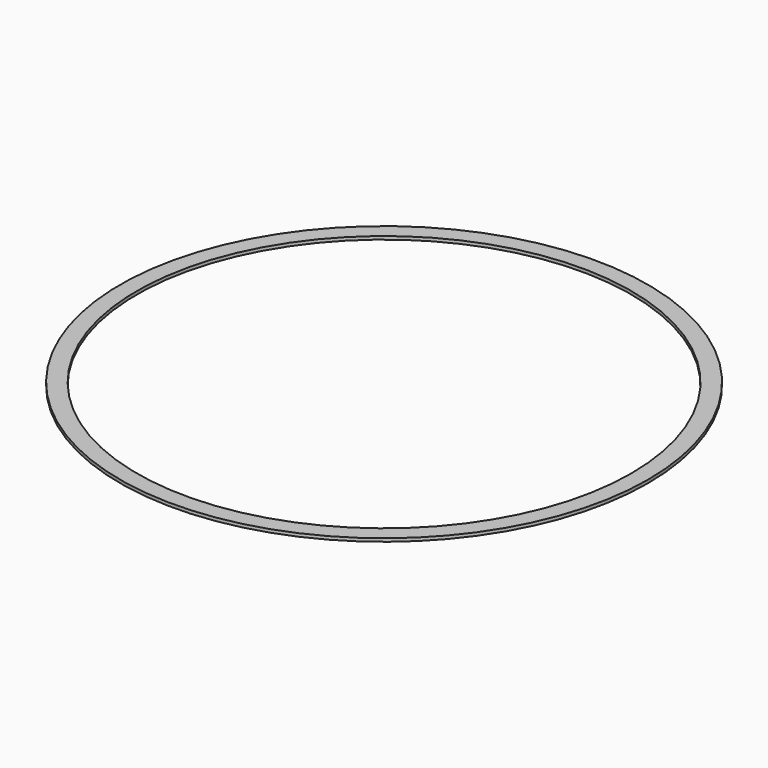
from build123d import *

# Parameters (mm, degrees)
F0_R     = 398.71523
F0_R_2   = 373.31523
F1_DEPTH = 4.7625


# Not quite as in the source:
# - a length typed as a fraction of an inch, garbled in the dataset ("3 / 203.2 mm" for 3/8 in), is restored


with BuildPart() as f1:
    # F0 (on Top) → F1 (new body)
    with BuildSketch(Plane.XY):
        Circle(F0_R)
        Circle(F0_R_2, mode=Mode.SUBTRACT)
    extrude(amount=F1_DEPTH)


solid = f1.part
